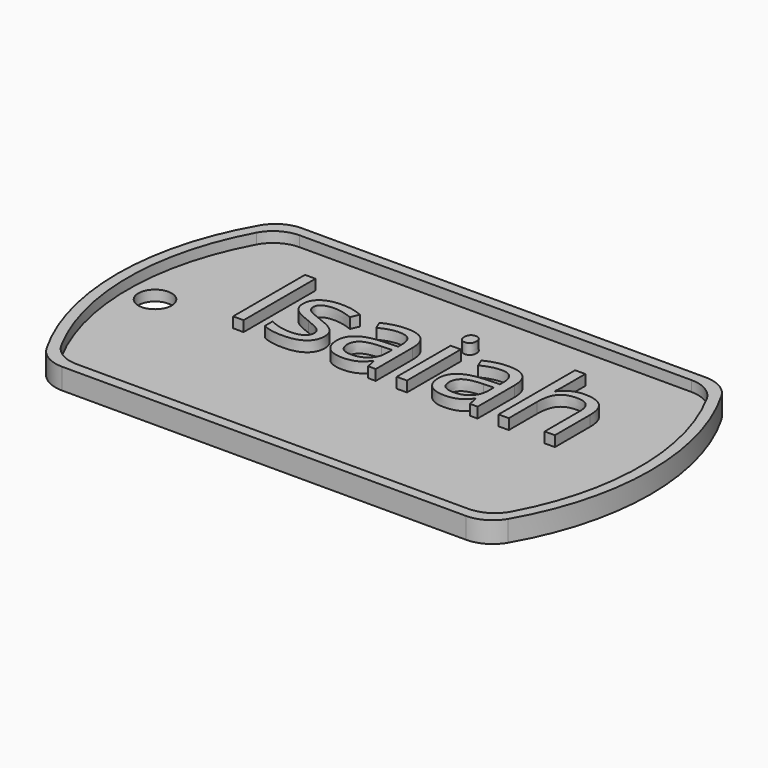
from build123d import *

# Parameters (mm, degrees)
F1_DEPTH     = 1
F3_DEPTH     = 1
F4_R         = 1.5875
F5_DEPTH     = 1
F6_TEXT_SIZE = 11.996505782
F7_DEPTH     = 1


# Not quite as in the source:
# - Text() gives the source's letters only with a copy of the font that has no kerning and outlines rounded to 1/6400 em; it was checked with that copy


with BuildPart() as f1:
    # F0 (on Top) → F1 (new body)
    with BuildSketch(Plane.XY):
        with BuildLine():
            ThreePointArc((-19.2474145991, 14.2875), (-20.8349145991, 13.862130657), (-21.9970452561, 12.7))
            ThreePointArc((-21.9970452561, 12.7), (-25.4, 0), (-21.9970452561, -12.7))
            ThreePointArc((-21.9970452561, -12.7), (-20.8349145991, -13.862130657), (-19.2474145991, -14.2875))
            Line((-19.2474145991, -14.2875), (19.2474145991, -14.2875))
            ThreePointArc((19.2474145991, -14.2875), (20.8349145991, -13.862130657), (21.9970452561, -12.7))
            ThreePointArc((21.9970452561, -12.7), (25.4, 0), (21.9970452561, 12.7))
            ThreePointArc((21.9970452561, 12.7), (20.8349145991, 13.862130657), (19.2474145991, 14.2875))
            Line((19.2474145991, 14.2875), (-19.2474145991, 14.2875))
        make_face()
    extrude(amount=F1_DEPTH)

    # F2 (on face) → F3 (join)
    with BuildSketch(Plane.XY.offset(1)):
        with BuildLine():
            Line((19.2474145991, 14.2875), (-19.2474145991, 14.2875))
            ThreePointArc((-19.2474145991, 14.2875), (-20.8349145991, 13.862130657), (-21.9970452561, 12.7))
            ThreePointArc((-21.9970452561, 12.7), (-25.4, 0), (-21.9970452561, -12.7))
            ThreePointArc((-21.9970452561, -12.7), (-20.8349145991, -13.862130657), (-19.2474145991, -14.2875))
            Line((-19.2474145991, -14.2875), (19.2474145991, -14.2875))
            ThreePointArc((19.2474145991, -14.2875), (20.8349145991, -13.862130657), (21.9970452561, -12.7))
            ThreePointArc((21.9970452561, -12.7), (25.4, 0), (21.9970452561, 12.7))
            ThreePointArc((21.9970452561, 12.7), (20.8349145991, 13.862130657), (19.2474145991, 14.2875))
        make_face()
        with BuildLine():
            ThreePointArc((-21.4526124879, 11.6252061249), (-20.2856017842, 12.8404540819), (-18.6611352482, 13.2875))
            Line((-18.6611352482, 13.2875), (18.6611352482, 13.2875))
            ThreePointArc((18.6611352482, 13.2875), (20.2856017842, 12.8404540819), (21.4526124879, 11.6252061249))
            ThreePointArc((21.4526124879, 11.6252061249), (24.4, 0), (21.4526124879, -11.6252061249))
            ThreePointArc((21.4526124879, -11.6252061249), (20.2856017842, -12.8404540819), (18.6611352482, -13.2875))
            Line((18.6611352482, -13.2875), (-18.6611352482, -13.2875))
            ThreePointArc((-18.6611352482, -13.2875), (-20.2856017842, -12.8404540819), (-21.4526124879, -11.6252061249))
            ThreePointArc((-21.4526124879, -11.6252061249), (-24.4, 0), (-21.4526124879, 11.6252061249))
        make_face(mode=Mode.SUBTRACT)
    extrude(amount=F3_DEPTH)

    # F4 (on face) → F5 (cut)
    with BuildSketch(Plane.XY.offset(1)):
        with Locations((-21.821282804, 0)):
            Circle(F4_R)
    extrude(amount=-F5_DEPTH, mode=Mode.SUBTRACT)

    # F6 (on face) → F7 (join)
    with BuildSketch(Plane.XY.offset(1)):
        with Locations((-15.5559327686, 0)):
            Text('Isaiah', F6_TEXT_SIZE, font='Open Sans', text_align=(TextAlign.LEFT, TextAlign.BOTTOM))
    extrude(amount=F7_DEPTH)


solid = f1.part
